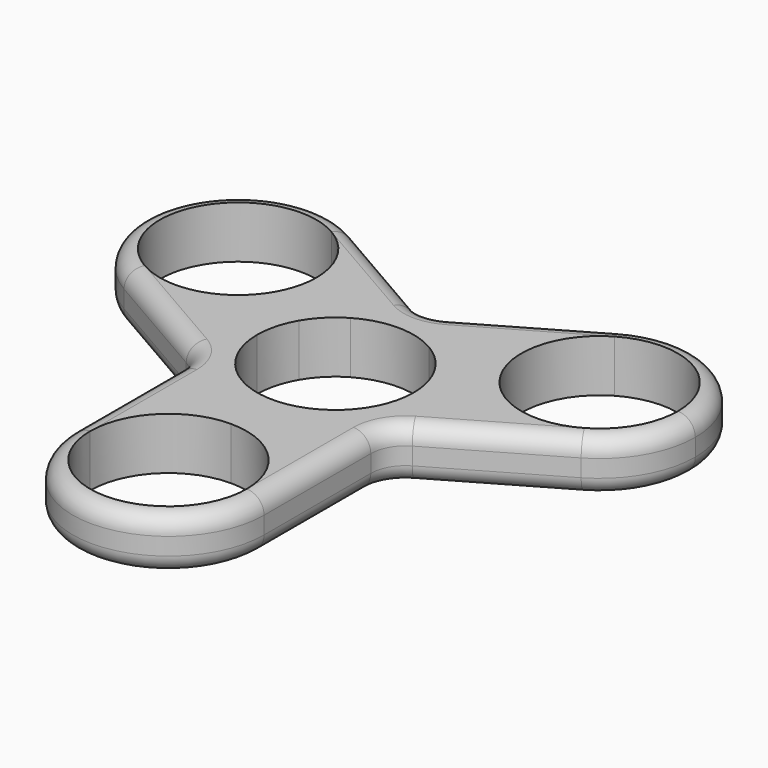
from build123d import *

# Parameters (mm, degrees)
F1_DEPTH = 7.62
F2_R     = 5.08
F3_R     = 2.53999


# Not quite as in the source:
# - a fillet or chamfer is up to 0.001 mm smaller than in the source, because OpenCascade refuses the exact size
# - a feature names something its author has since deleted; it is built from what else it names


with BuildPart() as f1:
    # F0 (on Top) → F1 (new body)
    with BuildSketch(Plane.XY):
        with BuildLine():
            Line((5.715, 9.8986703653), (6.985, 12.0983748909))
            ThreePointArc((6.985, 12.0983748909), (0, 13.97), (-6.985, 12.0983748909))
            Line((-6.985, 12.0983748909), (-5.715, 9.8986703653))
            ThreePointArc((-5.715, 9.8986703653), (0, 11.43), (5.715, 9.8986703653))
        make_face()
        with BuildLine():
            Line((0, 16.1311665212), (6.985, 12.0983748909))
            ThreePointArc((6.985, 12.0983748909), (9.8782817332, 9.8782817332), (12.0983748909, 6.985))
            Line((12.0983748909, 6.985), (14.2980794165, 8.255))
            ThreePointArc((14.2980794165, 8.255), (12.9024705141, 18.8557020601), (19.4114543073, 27.3383748909))
            Line((19.4114543073, 27.3383748909), (0, 16.1311665212))
        make_face()
        with BuildLine():
            ThreePointArc((-6.985, 12.0983748909), (0, 13.97), (6.985, 12.0983748909))
            Line((6.985, 12.0983748909), (0, 16.1311665212))
            Line((0, 16.1311665212), (-6.985, 12.0983748909))
        make_face()
        with BuildLine():
            ThreePointArc((12.0983748909, 6.985), (9.8782817332, 9.8782817332), (6.985, 12.0983748909))
            Line((6.985, 12.0983748909), (5.715, 9.8986703653))
            ThreePointArc((5.715, 9.8986703653), (8.082230509, 8.082230509), (9.8986703653, 5.715))
            Line((9.8986703653, 5.715), (12.0983748909, 6.985))
        make_face()
        with BuildLine():
            Line((-5.715, 9.8986703653), (-6.985, 12.0983748909))
            ThreePointArc((-6.985, 12.0983748909), (-9.8782817332, 9.8782817332), (-12.0983748909, 6.985))
            Line((-12.0983748909, 6.985), (-9.8986703653, 5.715))
            ThreePointArc((-9.8986703653, 5.715), (-8.082230509, 8.082230509), (-5.715, 9.8986703653))
        make_face()
        with BuildLine():
            ThreePointArc((-12.0983748909, 6.985), (-9.8782817332, 9.8782817332), (-6.985, 12.0983748909))
            Line((-6.985, 12.0983748909), (0, 16.1311665212))
            Line((0, 16.1311665212), (-19.4114543073, 27.3383748909))
            ThreePointArc((-19.4114543073, 27.3383748909), (-14.2980794165, 22.225), (-12.4264543073, 15.24))
            ThreePointArc((-12.4264543073, 15.24), (-12.9024705141, 11.6242979399), (-14.2980794165, 8.255))
            Line((-14.2980794165, 8.255), (-12.0983748909, 6.985))
        make_face()
        with BuildLine():
            Line((14.2980794165, 8.255), (12.0983748909, 6.985))
            ThreePointArc((12.0983748909, 6.985), (13.4939837933, 3.6157020601), (13.97, 0))
            Line((13.97, 0), (13.97, -8.0655832606))
            Line((13.97, -8.0655832606), (33.3814543073, 3.1416251091))
            ThreePointArc((33.3814543073, 3.1416251091), (22.7807522473, 1.7460162067), (14.2980794165, 8.255))
        make_face()
        with BuildLine():
            ThreePointArc((13.97, 0), (13.4939837933, 3.6157020601), (12.0983748909, 6.985))
            Line((12.0983748909, 6.985), (9.8986703653, 5.715))
            ThreePointArc((9.8986703653, 5.715), (11.0405321945, 2.9583016855), (11.43, 0))
            Line((11.43, 0), (13.97, 0))
        make_face()
        with BuildLine():
            Line((-9.8986703653, 5.715), (-12.0983748909, 6.985))
            ThreePointArc((-12.0983748909, 6.985), (-13.4939837933, 3.6157020601), (-13.97, 0))
            Line((-13.97, 0), (-11.43, 0))
            ThreePointArc((-11.43, 0), (-11.0405321945, 2.9583016855), (-9.8986703653, 5.715))
        make_face()
        with BuildLine():
            ThreePointArc((-13.97, 0), (-13.4939837933, 3.6157020601), (-12.0983748909, 6.985))
            Line((-12.0983748909, 6.985), (-14.2980794165, 8.255))
            ThreePointArc((-14.2980794165, 8.255), (-22.7807522473, 1.7460162067), (-33.3814543073, 3.1416251091))
            Line((-33.3814543073, 3.1416251091), (-13.97, -8.0655832606))
            Line((-13.97, -8.0655832606), (-13.97, 0))
        make_face()
        with BuildLine():
            Line((13.97, -8.0655832606), (13.97, 0))
            ThreePointArc((13.97, 0), (12.0983748909, -6.985), (6.985, -12.0983748909))
            Line((6.985, -12.0983748909), (13.97, -8.0655832606))
        make_face()
        with BuildLine():
            ThreePointArc((6.985, -12.0983748909), (12.0983748909, -6.985), (13.97, 0))
            Line((13.97, 0), (11.43, 0))
            ThreePointArc((11.43, 0), (9.8986703653, -5.715), (5.715, -9.8986703653))
            Line((5.715, -9.8986703653), (6.985, -12.0983748909))
        make_face()
        with BuildLine():
            Line((16.4977839421, 9.525), (14.2980794165, 8.255))
            ThreePointArc((14.2980794165, 8.255), (22.7807522473, 1.7460162067), (33.3814543073, 3.1416251091))
            Line((33.3814543073, 3.1416251091), (32.1114543073, 5.3413296347))
            ThreePointArc((32.1114543073, 5.3413296347), (23.4381526218, 4.1994678055), (16.4977839421, 9.525))
        make_face()
        with BuildLine():
            ThreePointArc((19.4114543073, 27.3383748909), (12.9024705141, 18.8557020601), (14.2980794165, 8.255))
            Line((14.2980794165, 8.255), (16.4977839421, 9.525))
            ThreePointArc((16.4977839421, 9.525), (15.3559221129, 18.1983016855), (20.6814543073, 25.1386703653))
            Line((20.6814543073, 25.1386703653), (19.4114543073, 27.3383748909))
        make_face()
        with BuildLine():
            ThreePointArc((40.3664543073, 15.24), (33.3814543073, 27.3383748909), (19.4114543073, 27.3383748909))
            Line((19.4114543073, 27.3383748909), (20.6814543073, 25.1386703653))
            ThreePointArc((20.6814543073, 25.1386703653), (32.1114543073, 25.1386703653), (37.8264543073, 15.24))
            ThreePointArc((37.8264543073, 15.24), (36.2951246726, 9.525), (32.1114543073, 5.3413296347))
            Line((32.1114543073, 5.3413296347), (33.3814543073, 3.1416251091))
            ThreePointArc((33.3814543073, 3.1416251091), (38.4948291982, 8.255), (40.3664543073, 15.24))
        make_face()
        with BuildLine():
            Line((-20.6814543073, 25.1386703653), (-19.4114543073, 27.3383748909))
            ThreePointArc((-19.4114543073, 27.3383748909), (-38.4948291982, 22.225), (-33.3814543073, 3.1416251091))
            Line((-33.3814543073, 3.1416251091), (-32.1114543073, 5.3413296347))
            ThreePointArc((-32.1114543073, 5.3413296347), (-36.2951246726, 20.955), (-20.6814543073, 25.1386703653))
        make_face()
        with BuildLine():
            ThreePointArc((-12.4264543073, 15.24), (-14.2980794165, 22.225), (-19.4114543073, 27.3383748909))
            Line((-19.4114543073, 27.3383748909), (-20.6814543073, 25.1386703653))
            ThreePointArc((-20.6814543073, 25.1386703653), (-16.4977839421, 20.955), (-14.9664543073, 15.24))
            ThreePointArc((-14.9664543073, 15.24), (-15.3559221129, 12.2816983145), (-16.4977839421, 9.525))
            Line((-16.4977839421, 9.525), (-14.2980794165, 8.255))
            ThreePointArc((-14.2980794165, 8.255), (-12.9024705141, 11.6242979399), (-12.4264543073, 15.24))
        make_face()
        with BuildLine():
            Line((-11.43, 0), (-13.97, 0))
            ThreePointArc((-13.97, 0), (-12.0983748909, -6.985), (-6.985, -12.0983748909))
            Line((-6.985, -12.0983748909), (-5.715, -9.8986703653))
            ThreePointArc((-5.715, -9.8986703653), (-9.8986703653, -5.715), (-11.43, 0))
        make_face()
        with BuildLine():
            ThreePointArc((-6.985, -12.0983748909), (-12.0983748909, -6.985), (-13.97, 0))
            Line((-13.97, 0), (-13.97, -8.0655832606))
            Line((-13.97, -8.0655832606), (-6.985, -12.0983748909))
        make_face()
        with BuildLine():
            ThreePointArc((-33.3814543073, 3.1416251091), (-22.7807522473, 1.7460162067), (-14.2980794165, 8.255))
            Line((-14.2980794165, 8.255), (-16.4977839421, 9.525))
            ThreePointArc((-16.4977839421, 9.525), (-23.4381526218, 4.1994678055), (-32.1114543073, 5.3413296347))
            Line((-32.1114543073, 5.3413296347), (-33.3814543073, 3.1416251091))
        make_face()
        with BuildLine():
            Line((13.97, -8.0655832606), (6.985, -12.0983748909))
            ThreePointArc((6.985, -12.0983748909), (3.6157020601, -13.4939837933), (0, -13.97))
            Line((0, -13.97), (0, -16.51))
            ThreePointArc((0, -16.51), (9.8782817332, -20.6017182668), (13.97, -30.48))
            Line((13.97, -30.48), (13.97, -8.0655832606))
        make_face()
        with BuildLine():
            ThreePointArc((0, -13.97), (3.6157020601, -13.4939837933), (6.985, -12.0983748909))
            Line((6.985, -12.0983748909), (5.715, -9.8986703653))
            ThreePointArc((5.715, -9.8986703653), (2.9583016855, -11.0405321945), (0, -11.43))
            Line((0, -11.43), (0, -13.97))
        make_face()
        with BuildLine():
            Line((0, -13.97), (0, -11.43))
            ThreePointArc((0, -11.43), (-2.9583016855, -11.0405321945), (-5.715, -9.8986703653))
            Line((-5.715, -9.8986703653), (-6.985, -12.0983748909))
            ThreePointArc((-6.985, -12.0983748909), (-3.6157020601, -13.4939837933), (0, -13.97))
        make_face()
        with BuildLine():
            ThreePointArc((0, -13.97), (-3.6157020601, -13.4939837933), (-6.985, -12.0983748909))
            Line((-6.985, -12.0983748909), (-13.97, -8.0655832606))
            Line((-13.97, -8.0655832606), (-13.97, -30.48))
            ThreePointArc((-13.97, -30.48), (-9.8782817332, -20.6017182668), (0, -16.51))
            Line((0, -16.51), (0, -13.97))
        make_face()
        with BuildLine():
            Line((11.43, -30.48), (13.97, -30.48))
            ThreePointArc((13.97, -30.48), (9.8782817332, -20.6017182668), (0, -16.51))
            Line((0, -16.51), (0, -19.05))
            ThreePointArc((0, -19.05), (8.082230509, -22.397769491), (11.43, -30.48))
        make_face()
        with BuildLine():
            ThreePointArc((-13.97, -30.48), (0, -44.45), (13.97, -30.48))
            Line((13.97, -30.48), (11.43, -30.48))
            ThreePointArc((11.43, -30.48), (0, -41.91), (-11.43, -30.48))
            Line((-11.43, -30.48), (-13.97, -30.48))
        make_face()
        with BuildLine():
            ThreePointArc((0, -16.51), (-9.8782817332, -20.6017182668), (-13.97, -30.48))
            Line((-13.97, -30.48), (-11.43, -30.48))
            ThreePointArc((-11.43, -30.48), (-8.082230509, -22.397769491), (0, -19.05))
            Line((0, -19.05), (0, -16.51))
        make_face()
    extrude(amount=F1_DEPTH)

    # F2
    f2_edges = [f1.edges().sort_by_distance(p)[0] for p in [
        (0, 16.131167, 3.81),
        (13.97, -8.065583, 3.81),
        (-13.97, -8.065583, 3.81),
    ]]
    fillet(f2_edges, radius=F2_R)

    # F3 (radius 2.54 in the source; OpenCascade refuses exactly that, so slightly less here)
    f3_edges = [f1.edges().sort_by_distance(p)[0] for p in [
        (24.945727, -1.728744, 7.62),
        (14.650591, -8.458523, 7.62),
        (-13.97, -20.739261, 0),
        (10.975727, 22.468006, 0),
        (10.975727, 22.468006, 7.62),
        (0, 16.917045, 0),
        (38.494829, 22.225, 0),
        (-10.975727, 22.468006, 0),
        (24.945727, -1.728744, 0),
        (-38.494829, 22.225, 0),
        (14.650591, -8.458523, 0),
        (-24.945727, -1.728744, 0),
        (13.97, -20.739261, 0),
        (-14.650591, -8.458523, 0),
        (0, -44.45, 0),
        (0, 16.917045, 7.62),
        (38.494829, 22.225, 7.62),
        (-10.975727, 22.468006, 7.62),
        (-38.494829, 22.225, 7.62),
        (-24.945727, -1.728744, 7.62),
        (13.97, -20.739261, 7.62),
        (-14.650591, -8.458523, 7.62),
        (0, -44.45, 7.62),
        (-13.97, -20.739261, 7.62),
    ]]
    fillet(f3_edges, radius=F3_R)


solid = f1.part
